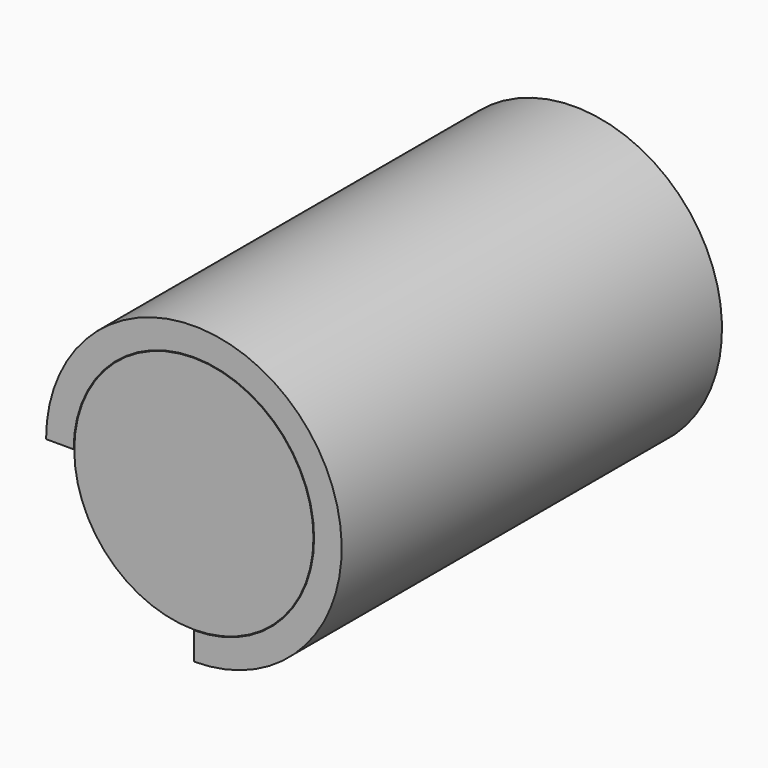
from build123d import *

# Parameters (mm, degrees)
F0_R      = 49.7360969104
F1_DEPTH  = 80
F2_R      = 40.4600824773
F3_DEPTH  = 90
F4_R      = 8.4494830611
F5_DEPTH  = 65
F7_R      = 40.2505245535
F8_DEPTH  = 30
F10_R     = 40.3514508638
F11_DEPTH = 5
F13_R     = 40.2465604933
F14_DEPTH = 30
F16_R     = 19.6314751685
F17_DEPTH = 50
F18_R     = 28.4934569002
F19_DEPTH = 25
F20_W     = 76.695650816
F20_H     = 61.7673955858
F21_DEPTH = 180
F23_R     = 12.0703792792
F24_DEPTH = 2.5


with BuildPart() as f1:
    # F0 (on Front) → F1 (new body, symmetric)
    with BuildSketch(Plane.XZ):
        Circle(F0_R)
    extrude(amount=F1_DEPTH, both=True)

    # F2 (on Front) → F3 (cut, symmetric)
    with BuildSketch(Plane.XZ):
        Circle(F2_R)
    extrude(amount=F3_DEPTH, both=True, mode=Mode.SUBTRACT)

    # F20 (on offset) → F21 (cut)
    with BuildSketch(Plane.XZ.offset(-80)):
        with Locations((-38.347825408, -30.8836977929)):
            Rectangle(F20_W, F20_H)
    extrude(amount=F21_DEPTH, mode=Mode.SUBTRACT)


with BuildPart() as f5:
    # F4 (on Front) → F5 (new body, symmetric)
    with BuildSketch(Plane.XZ):
        Circle(F4_R)
    extrude(amount=F5_DEPTH, both=True)


with BuildPart() as f8:
    # F7 (on offset) → F8 (new body)
    with BuildSketch(Plane.XZ.offset(80)):
        Circle(F7_R)
    extrude(amount=-F8_DEPTH)


with BuildPart() as f11:
    # F10 (on offset) → F11 (new body)
    with BuildSketch(Plane.XZ.offset(50)):
        Circle(F10_R)
    extrude(amount=-F11_DEPTH)


with BuildPart() as f14:
    # F13 (on offset) → F14 (new body)
    with BuildSketch(Plane.XZ.offset(-80)):
        Circle(F13_R)
    extrude(amount=F14_DEPTH)

    # F18 (on offset) → F19 (cut)
    with BuildSketch(Plane.XZ.offset(-80)):
        Circle(F18_R)
    extrude(amount=F19_DEPTH, mode=Mode.SUBTRACT)


with BuildPart() as f17:
    # F16 (on offset) → F17 (new body)
    with BuildSketch(Plane.XZ.offset(-50)):
        Circle(F16_R)
    extrude(amount=F17_DEPTH)


with BuildPart() as f24:
    # F23 (on offset) → F24 (new body)
    with BuildSketch(Plane.XZ.offset(45)):
        with Locations((0.1020442141, 0.0310293544)):
            Circle(F23_R)
    extrude(amount=-F24_DEPTH)


solid = Compound([f1.part, f5.part, f8.part, f11.part, f14.part, f17.part, f24.part])
